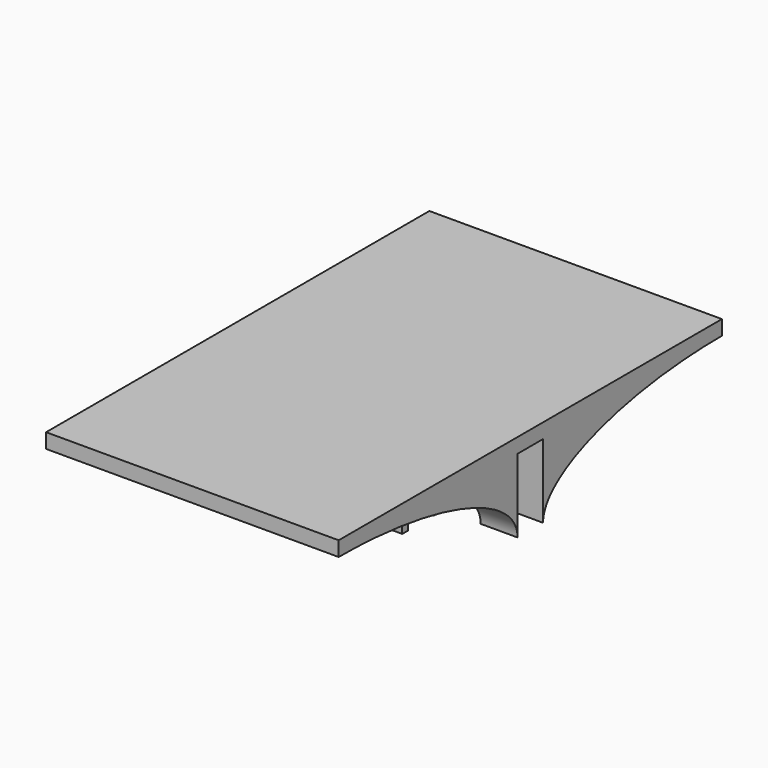
from build123d import *

# Parameters (mm, degrees)
F0_W             = 39.7
F0_H             = 65
F1_DEPTH         = 2
F3_DEPTH         = 5
F3_COPIES2_COUNT = 2
F5_DEPTH         = 5
F6_R             = 1.8
F7_DEPTH         = 35.6610001


# Not quite as in the source:
# - a pattern or mirror of a feature is missing from the dataset's text; its kind, count and spacing are read off the source's solid


with BuildPart() as f1:
    # F0 (on Top) → F1 (new body)
    with BuildSketch(Plane.XY):
        Rectangle(F0_W, F0_H)
    extrude(amount=F1_DEPTH)

    # F2 (on face) → F3 (join)
    with BuildSketch(Plane.YZ.offset(19.85)):
        with BuildLine():
            add(Edge.make_bspline(
                [(-2.16, -10), (-2.16, 0), (-32.5, 0)],
                knots=[0, 0, 0, 1.5707963268, 1.5707963268, 1.5707963268], degree=2, weights=[1, 0.7071067812, 1]))
            Line((-2.16, -10), (-2.16, 0))
            Line((-2.16, 0), (-32.5, 0))
        make_face()
    f3 = extrude(amount=-F3_DEPTH)

    # F3_copies: F3 across plane
    add(f3.mirror(Plane.ZX))

    # F3_copies1: F3 across plane
    add(f3.mirror(Plane(origin=(0, 0, 0), x_dir=(0, 0, -1), z_dir=(-1, 0, 0))))

    # F3_copies2: F3 ×2 about axis
    f3_copies2_axis = Axis((0, 0, 0), (0, 0, 1))
    for i in range(1, F3_COPIES2_COUNT):
        add(f3.rotate(f3_copies2_axis, i * 360 / F3_COPIES2_COUNT))

    # F4 (on Right) → F5 (join, symmetric)
    with BuildSketch(Plane.YZ):
        Polygon((-2.16, -14), (-2.16, -10), (-2.16, 0), (-3.16, 0), (-3.16, -14), align=None)
    f5 = extrude(amount=F5_DEPTH, both=True)

    # F5_copies: F5 across plane
    add(f5.mirror(Plane.ZX))

    # F6 (on face) → F7 (cut, through all)
    with BuildSketch(Plane.XZ.offset(3.16)):
        with Locations((0, -8)):
            Circle(F6_R)
    extrude(amount=-F7_DEPTH, mode=Mode.SUBTRACT)


solid = f1.part
